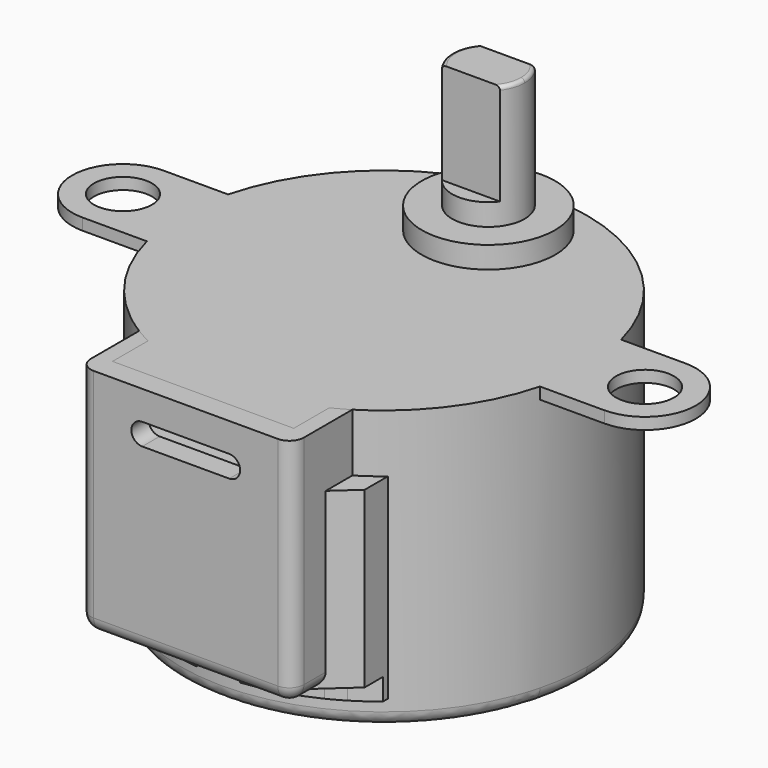
from build123d import *
from build123d import SkipClean  # not in build123d's __all__

# Parameters (mm, degrees)
F0_R      = 2
F0_R_2    = 4.6
F1_DEPTH  = 0.8
F2_DEPTH  = 19.3
F3_R      = 1
F4_DEPTH  = 1.5
F7_DEPTH  = 4
F8_DEPTH  = 12
F9_DEPTH  = 13.5
F11_R     = 1
F14_DEPTH = 3
F15_DEPTH = 3
F16_DEPTH = 10
F17_R     = 0.25


with BuildPart() as f1:
    # F0 (on Top) → F1 (new body)
    with BuildSketch(Plane.XY):
        with BuildLine():
            ThreePointArc((-13.5554417117, -3.5), (-14, 0), (-13.5554417117, 3.5))
            Line((-13.5554417117, 3.5), (-18, 3.5))
            ThreePointArc((-18, 3.5), (-21.5, 0), (-18, -3.5))
            Line((-18, -3.5), (-13.5554417117, -3.5))
        make_face()
        with Locations((-18, 0)):
            Circle(F0_R, mode=Mode.SUBTRACT)
        with BuildLine():
            ThreePointArc((13.5554417117, -3.5), (13.8884157477, -1.7640600948), (14, 0))
            ThreePointArc((14, 0), (13.8884157477, 1.7640600948), (13.5554417117, 3.5))
            ThreePointArc((13.5554417117, 3.5), (0, 14), (-13.5554417117, 3.5))
            ThreePointArc((-13.5554417117, 3.5), (-14, 0), (-13.5554417117, -3.5))
            ThreePointArc((-13.5554417117, -3.5), (-11.7352824288, -7.6343399398), (-8.6933517225, -10.9738614821))
            ThreePointArc((-8.6933517225, -10.9738614821), (-8.0354789523, -11.4643394056), (-7.35, -11.9154311714))
            ThreePointArc((-7.35, -11.9154311714), (-6.8068823867, -12.2338200156), (-6.25, -12.5274698164))
            ThreePointArc((-6.25, -12.5274698164), (-3.937003937, -13.4350288425), (-1.5, -13.9194109071))
            ThreePointArc((-1.5, -13.9194109071), (0, -14), (1.5, -13.9194109071))
            ThreePointArc((1.5, -13.9194109071), (3.937003937, -13.4350288425), (6.25, -12.5274698164))
            ThreePointArc((6.25, -12.5274698164), (6.8068823867, -12.2338200156), (7.35, -11.9154311714))
            ThreePointArc((7.35, -11.9154311714), (8.1473851159, -11.3850830376), (8.9066482775, -10.8014636259))
            ThreePointArc((8.9066482775, -10.8014636259), (11.8094967903, -7.5190282324), (13.5554417117, -3.5))
        make_face()
        with Locations((0, 9)):
            Circle(F0_R_2, mode=Mode.SUBTRACT)
        with BuildLine():
            ThreePointArc((13.5554417117, 3.5), (13.8884157477, 1.7640600948), (14, 0))
            ThreePointArc((14, 0), (13.8884157477, -1.7640600948), (13.5554417117, -3.5))
            Line((13.5554417117, -3.5), (18, -3.5))
            ThreePointArc((18, -3.5), (21.5, 0), (18, 3.5))
            Line((18, 3.5), (13.5554417117, 3.5))
        make_face()
        with Locations((18, 0)):
            Circle(F0_R, mode=Mode.SUBTRACT)
        with Locations((0, 9)):
            Circle(F0_R_2)
        with BuildLine():
            ThreePointArc((2, 10.5), (2.3717082451, 9.790569415), (2.5, 9))
            ThreePointArc((2.5, 9), (2.3717082451, 8.209430585), (2, 7.5))
            ThreePointArc((2, 7.5), (0, 6.5), (-2, 7.5))
            ThreePointArc((-2, 7.5), (-2.5, 9), (-2, 10.5))
            ThreePointArc((-2, 10.5), (0, 11.5), (2, 10.5))
        make_face(mode=Mode.SUBTRACT)
        with BuildLine():
            ThreePointArc((2, 7.5), (2.3717082451, 8.209430585), (2.5, 9))
            ThreePointArc((2.5, 9), (2.3717082451, 9.790569415), (2, 10.5))
            Line((2, 10.5), (-2, 10.5))
            ThreePointArc((-2, 10.5), (-2.5, 9), (-2, 7.5))
            Line((-2, 7.5), (2, 7.5))
        make_face()
        with BuildLine():
            ThreePointArc((-1.5, -13.9194109071), (-3.937003937, -13.4350288425), (-6.25, -12.5274698164))
            Line((-6.25, -12.5274698164), (-6.25, -12.9263565834))
            ThreePointArc((-6.25, -12.9263565834), (-3.9357520983, -13.8246688211), (-1.5, -14.3040642142))
            Line((-1.5, -14.3040642142), (-1.5, -13.9194109071))
        make_face()
        with BuildLine():
            Line((1.5, -14.3040642142), (1.5, -13.9194109071))
            ThreePointArc((1.5, -13.9194109071), (0, -14), (-1.5, -13.9194109071))
            Line((-1.5, -13.9194109071), (-1.5, -14.3040642142))
            ThreePointArc((-1.5, -14.3040642142), (-3.9357520983, -13.8246688211), (-6.25, -12.9263565834))
            Line((-6.25, -12.9263565834), (-6.25, -15.591))
            Line((-6.25, -15.591), (6.25, -15.591))
            Line((6.25, -15.591), (6.25, -12.9263565834))
            ThreePointArc((6.25, -12.9263565834), (3.9357520983, -13.8246688211), (1.5, -14.3040642142))
        make_face()
        with BuildLine():
            Line((1.5, -14.3040642142), (1.5, -13.9194109071))
            ThreePointArc((1.5, -13.9194109071), (0, -14), (-1.5, -13.9194109071))
            Line((-1.5, -13.9194109071), (-1.5, -14.3040642142))
            ThreePointArc((-1.5, -14.3040642142), (-3.9357520983, -13.8246688211), (-6.25, -12.9263565834))
            Line((-6.25, -12.9263565834), (-6.25, -15.591))
            Line((-6.25, -15.591), (6.25, -15.591))
            Line((6.25, -15.591), (6.25, -12.9263565834))
            ThreePointArc((6.25, -12.9263565834), (3.9357520983, -13.8246688211), (1.5, -14.3040642142))
        make_face()
        with BuildLine():
            Line((6.25, -12.9263565834), (6.25, -12.5274698164))
            ThreePointArc((6.25, -12.5274698164), (3.937003937, -13.4350288425), (1.5, -13.9194109071))
            Line((1.5, -13.9194109071), (1.5, -14.3040642142))
            ThreePointArc((1.5, -14.3040642142), (3.9357520983, -13.8246688211), (6.25, -12.9263565834))
        make_face()
        with BuildLine():
            Line((-2, 10.5), (2, 10.5))
            ThreePointArc((2, 10.5), (0, 11.5), (-2, 10.5))
        make_face()
        with BuildLine():
            ThreePointArc((-2, 7.5), (0, 6.5), (2, 7.5))
            Line((2, 7.5), (-2, 7.5))
        make_face()
    extrude(amount=-F1_DEPTH)

    # F0 (on Top) → F2 (join)
    with BuildSketch(Plane.XY):
        with BuildLine():
            ThreePointArc((13.5554417117, -3.5), (13.8884157477, -1.7640600948), (14, 0))
            ThreePointArc((14, 0), (13.8884157477, 1.7640600948), (13.5554417117, 3.5))
            ThreePointArc((13.5554417117, 3.5), (0, 14), (-13.5554417117, 3.5))
            ThreePointArc((-13.5554417117, 3.5), (-14, 0), (-13.5554417117, -3.5))
            ThreePointArc((-13.5554417117, -3.5), (-11.7352824288, -7.6343399398), (-8.6933517225, -10.9738614821))
            ThreePointArc((-8.6933517225, -10.9738614821), (-8.0354789523, -11.4643394056), (-7.35, -11.9154311714))
            ThreePointArc((-7.35, -11.9154311714), (-6.8068823867, -12.2338200156), (-6.25, -12.5274698164))
            ThreePointArc((-6.25, -12.5274698164), (-3.937003937, -13.4350288425), (-1.5, -13.9194109071))
            ThreePointArc((-1.5, -13.9194109071), (0, -14), (1.5, -13.9194109071))
            ThreePointArc((1.5, -13.9194109071), (3.937003937, -13.4350288425), (6.25, -12.5274698164))
            ThreePointArc((6.25, -12.5274698164), (6.8068823867, -12.2338200156), (7.35, -11.9154311714))
            ThreePointArc((7.35, -11.9154311714), (8.1473851159, -11.3850830376), (8.9066482775, -10.8014636259))
            ThreePointArc((8.9066482775, -10.8014636259), (11.8094967903, -7.5190282324), (13.5554417117, -3.5))
        make_face()
        with Locations((0, 9)):
            Circle(F0_R_2, mode=Mode.SUBTRACT)
        with Locations((0, 9)):
            Circle(F0_R_2)
        with BuildLine():
            ThreePointArc((2, 10.5), (2.3717082451, 9.790569415), (2.5, 9))
            ThreePointArc((2.5, 9), (2.3717082451, 8.209430585), (2, 7.5))
            ThreePointArc((2, 7.5), (0, 6.5), (-2, 7.5))
            ThreePointArc((-2, 7.5), (-2.5, 9), (-2, 10.5))
            ThreePointArc((-2, 10.5), (0, 11.5), (2, 10.5))
        make_face(mode=Mode.SUBTRACT)
        with BuildLine():
            ThreePointArc((2, 7.5), (2.3717082451, 8.209430585), (2.5, 9))
            ThreePointArc((2.5, 9), (2.3717082451, 9.790569415), (2, 10.5))
            Line((2, 10.5), (-2, 10.5))
            ThreePointArc((-2, 10.5), (-2.5, 9), (-2, 7.5))
            Line((-2, 7.5), (2, 7.5))
        make_face()
        with BuildLine():
            Line((-2, 10.5), (2, 10.5))
            ThreePointArc((2, 10.5), (0, 11.5), (-2, 10.5))
        make_face()
        with BuildLine():
            ThreePointArc((-2, 7.5), (0, 6.5), (2, 7.5))
            Line((2, 7.5), (-2, 7.5))
        make_face()
    extrude(amount=-F2_DEPTH)

    # F3
    f3_edges = [f1.edges().sort_by_distance(p)[0] for p in [
        (13.555442, 3.5, -19.3),
    ]]
    fillet(f3_edges, radius=F3_R)

    # F0 (on Top) → F4 (join)
    with BuildSketch(Plane.XY):
        with Locations((0, 9)):
            Circle(F0_R_2)
        with BuildLine():
            ThreePointArc((2, 10.5), (2.3717082451, 9.790569415), (2.5, 9))
            ThreePointArc((2.5, 9), (2.3717082451, 8.209430585), (2, 7.5))
            ThreePointArc((2, 7.5), (0, 6.5), (-2, 7.5))
            ThreePointArc((-2, 7.5), (-2.5, 9), (-2, 10.5))
            ThreePointArc((-2, 10.5), (0, 11.5), (2, 10.5))
        make_face(mode=Mode.SUBTRACT)
    extrude(amount=F4_DEPTH)


with BuildPart() as f7:
    # F6 (on offset) → F7 (new body)
    with BuildSketch(Plane.XY.offset(-4)):
        with BuildLine():
            ThreePointArc((-6.25, -12.9263565834), (-6.8067194333, -12.6362058443), (-7.35, -12.3216105412))
            Line((-7.35, -12.3216105412), (-7.35, -14.2114134505))
            Line((-7.35, -14.2114134505), (-7.35, -17.091))
            Line((-7.35, -17.091), (7.35, -17.091))
            Line((7.35, -17.091), (7.35, -14.2114134505))
            Line((7.35, -14.2114134505), (7.35, -12.3216105412))
            ThreePointArc((7.35, -12.3216105412), (6.8067194333, -12.6362058443), (6.25, -12.9263565834))
            Line((6.25, -12.9263565834), (6.25, -15.591))
            Line((6.25, -15.591), (-6.25, -15.591))
            Line((-6.25, -15.591), (-6.25, -12.9263565834))
        make_face()
        with BuildLine():
            ThreePointArc((-6.25, -12.5274698164), (-6.8068823867, -12.2338200156), (-7.35, -11.9154311714))
            Line((-7.35, -11.9154311714), (-7.35, -12.3216105412))
            ThreePointArc((-7.35, -12.3216105412), (-6.8067194333, -12.6362058443), (-6.25, -12.9263565834))
            Line((-6.25, -12.9263565834), (-6.25, -12.5274698164))
        make_face()
        with BuildLine():
            Line((7.35, -12.3216105412), (7.35, -11.9154311714))
            ThreePointArc((7.35, -11.9154311714), (6.8068823867, -12.2338200156), (6.25, -12.5274698164))
            Line((6.25, -12.5274698164), (6.25, -12.9263565834))
            ThreePointArc((6.25, -12.9263565834), (6.8067194333, -12.6362058443), (7.35, -12.3216105412))
        make_face()
    extrude(amount=F7_DEPTH)

    # F6 (on offset) → F8 (join)
    with BuildSketch(Plane.XY.offset(-4)):
        with BuildLine():
            ThreePointArc((-6.25, -12.9263565834), (-6.8067194333, -12.6362058443), (-7.35, -12.3216105412))
            Line((-7.35, -12.3216105412), (-7.35, -14.2114134505))
            Line((-7.35, -14.2114134505), (-7.35, -17.091))
            Line((-7.35, -17.091), (7.35, -17.091))
            Line((7.35, -17.091), (7.35, -14.2114134505))
            Line((7.35, -14.2114134505), (7.35, -12.3216105412))
            ThreePointArc((7.35, -12.3216105412), (6.8067194333, -12.6362058443), (6.25, -12.9263565834))
            Line((6.25, -12.9263565834), (6.25, -15.591))
            Line((6.25, -15.591), (-6.25, -15.591))
            Line((-6.25, -15.591), (-6.25, -12.9263565834))
        make_face()
        with BuildLine():
            ThreePointArc((-1.5, -13.9194109071), (-3.937003937, -13.4350288425), (-6.25, -12.5274698164))
            Line((-6.25, -12.5274698164), (-6.25, -12.9263565834))
            ThreePointArc((-6.25, -12.9263565834), (-3.9357520983, -13.8246688211), (-1.5, -14.3040642142))
            Line((-1.5, -14.3040642142), (-1.5, -13.9194109071))
        make_face()
        with BuildLine():
            ThreePointArc((-6.25, -12.5274698164), (-6.8068823867, -12.2338200156), (-7.35, -11.9154311714))
            Line((-7.35, -11.9154311714), (-7.35, -12.3216105412))
            ThreePointArc((-7.35, -12.3216105412), (-6.8067194333, -12.6362058443), (-6.25, -12.9263565834))
            Line((-6.25, -12.9263565834), (-6.25, -12.5274698164))
        make_face()
        with BuildLine():
            ThreePointArc((-7.35, -11.9154311714), (-8.0354789523, -11.4643394056), (-8.6933517225, -10.9738614821))
            Line((-8.6933517225, -10.9738614821), (-8.6933517225, -11.3928156516))
            ThreePointArc((-8.6933517225, -11.3928156516), (-8.0351072557, -11.876639438), (-7.35, -12.3216105412))
            Line((-7.35, -12.3216105412), (-7.35, -11.9154311714))
        make_face()
        with BuildLine():
            ThreePointArc((-7.35, -12.3216105412), (-8.0351072557, -11.876639438), (-8.6933517225, -11.3928156516))
            Line((-8.6933517225, -11.3928156516), (-8.6933517225, -12.9738614821))
            Line((-8.6933517225, -12.9738614821), (-7.35, -14.2114134505))
            Line((-7.35, -14.2114134505), (-7.35, -12.3216105412))
        make_face()
        with BuildLine():
            Line((7.35, -12.3216105412), (7.35, -11.9154311714))
            ThreePointArc((7.35, -11.9154311714), (6.8068823867, -12.2338200156), (6.25, -12.5274698164))
            Line((6.25, -12.5274698164), (6.25, -12.9263565834))
            ThreePointArc((6.25, -12.9263565834), (6.8067194333, -12.6362058443), (7.35, -12.3216105412))
        make_face()
        with BuildLine():
            Line((8.9066482775, -11.2229927703), (8.9066482775, -10.8014636259))
            ThreePointArc((8.9066482775, -10.8014636259), (8.1473851159, -11.3850830376), (7.35, -11.9154311714))
            Line((7.35, -11.9154311714), (7.35, -12.3216105412))
            ThreePointArc((7.35, -12.3216105412), (8.146864032, -11.7985711133), (8.9066482775, -11.2229927703))
        make_face()
        with BuildLine():
            Line((8.9066482775, -12.8014636259), (8.9066482775, -11.2229927703))
            ThreePointArc((8.9066482775, -11.2229927703), (8.146864032, -11.7985711133), (7.35, -12.3216105412))
            Line((7.35, -12.3216105412), (7.35, -14.2114134505))
            Line((7.35, -14.2114134505), (8.9066482775, -12.8014636259))
        make_face()
        with BuildLine():
            Line((6.25, -12.9263565834), (6.25, -12.5274698164))
            ThreePointArc((6.25, -12.5274698164), (3.937003937, -13.4350288425), (1.5, -13.9194109071))
            Line((1.5, -13.9194109071), (1.5, -14.3040642142))
            ThreePointArc((1.5, -14.3040642142), (3.9357520983, -13.8246688211), (6.25, -12.9263565834))
        make_face()
        with BuildLine():
            ThreePointArc((1.5, -13.9194109071), (0, -14), (-1.5, -13.9194109071))
            Line((-1.5, -13.9194109071), (-1.5, -14.3040642142))
            ThreePointArc((-1.5, -14.3040642142), (-3.9357520983, -13.8246688211), (-6.25, -12.9263565834))
            Line((-6.25, -12.9263565834), (-6.25, -15.591))
            Line((-6.25, -15.591), (6.25, -15.591))
            Line((6.25, -15.591), (6.25, -12.9263565834))
            ThreePointArc((6.25, -12.9263565834), (3.9357520983, -13.8246688211), (1.5, -14.3040642142))
            Line((1.5, -14.3040642142), (1.5, -13.9194109071))
        make_face()
    extrude(amount=-F8_DEPTH)

    # F6 (on offset) → F9 (join)
    with BuildSketch(Plane.XY.offset(-4)):
        with BuildLine():
            ThreePointArc((-7.35, -11.9154311714), (-8.0354789523, -11.4643394056), (-8.6933517225, -10.9738614821))
            Line((-8.6933517225, -10.9738614821), (-8.6933517225, -11.3928156516))
            ThreePointArc((-8.6933517225, -11.3928156516), (-8.0351072557, -11.876639438), (-7.35, -12.3216105412))
            Line((-7.35, -12.3216105412), (-7.35, -11.9154311714))
        make_face()
        with BuildLine():
            ThreePointArc((-6.25, -12.5274698164), (-6.8068823867, -12.2338200156), (-7.35, -11.9154311714))
            Line((-7.35, -11.9154311714), (-7.35, -12.3216105412))
            ThreePointArc((-7.35, -12.3216105412), (-6.8067194333, -12.6362058443), (-6.25, -12.9263565834))
            Line((-6.25, -12.9263565834), (-6.25, -12.5274698164))
        make_face()
        with BuildLine():
            ThreePointArc((-1.5, -13.9194109071), (-3.937003937, -13.4350288425), (-6.25, -12.5274698164))
            Line((-6.25, -12.5274698164), (-6.25, -12.9263565834))
            ThreePointArc((-6.25, -12.9263565834), (-3.9357520983, -13.8246688211), (-1.5, -14.3040642142))
            Line((-1.5, -14.3040642142), (-1.5, -13.9194109071))
        make_face()
        with BuildLine():
            Line((6.25, -12.9263565834), (6.25, -12.5274698164))
            ThreePointArc((6.25, -12.5274698164), (3.937003937, -13.4350288425), (1.5, -13.9194109071))
            Line((1.5, -13.9194109071), (1.5, -14.3040642142))
            ThreePointArc((1.5, -14.3040642142), (3.9357520983, -13.8246688211), (6.25, -12.9263565834))
        make_face()
        with BuildLine():
            Line((7.35, -12.3216105412), (7.35, -11.9154311714))
            ThreePointArc((7.35, -11.9154311714), (6.8068823867, -12.2338200156), (6.25, -12.5274698164))
            Line((6.25, -12.5274698164), (6.25, -12.9263565834))
            ThreePointArc((6.25, -12.9263565834), (6.8067194333, -12.6362058443), (7.35, -12.3216105412))
        make_face()
        with BuildLine():
            Line((8.9066482775, -11.2229927703), (8.9066482775, -10.8014636259))
            ThreePointArc((8.9066482775, -10.8014636259), (8.1473851159, -11.3850830376), (7.35, -11.9154311714))
            Line((7.35, -11.9154311714), (7.35, -12.3216105412))
            ThreePointArc((7.35, -12.3216105412), (8.146864032, -11.7985711133), (8.9066482775, -11.2229927703))
        make_face()
    extrude(amount=-F9_DEPTH)

    # F10: union 

    # F11
    f11_edges = [f7.edges().sort_by_distance(p)[0] for p in [
        (-7.35, -17.091, -8),
        (0, -17.091, -16),
        (7.35, -17.091, -8),
        (-7.35, -15.651207, -16),
        (7.35, -15.651207, -16),
    ]]
    fillet(f11_edges, radius=F11_R)

    # F13 (on offset) → F14 (cut)
    with BuildSketch(Plane.XZ.offset(17.091)):
        with BuildLine():
            ThreePointArc((3, -3.5), (3.75, -2.75), (3, -2))
            Line((3, -2), (-3, -2))
            ThreePointArc((-3, -2), (-3.75, -2.75), (-3, -3.5))
            Line((-3, -3.5), (3, -3.5))
        make_face()
    extrude(amount=-F14_DEPTH, mode=Mode.SUBTRACT)


with BuildPart() as f15:
    # F0 (on Top) → F15 (new body)
    with BuildSketch(Plane.XY):
        with BuildLine():
            Line((-2, 10.5), (2, 10.5))
            ThreePointArc((2, 10.5), (0, 11.5), (-2, 10.5))
        make_face()
        with BuildLine():
            ThreePointArc((2, 7.5), (2.3717082451, 8.209430585), (2.5, 9))
            ThreePointArc((2.5, 9), (2.3717082451, 9.790569415), (2, 10.5))
            Line((2, 10.5), (-2, 10.5))
            ThreePointArc((-2, 10.5), (-2.5, 9), (-2, 7.5))
            Line((-2, 7.5), (2, 7.5))
        make_face()
        with BuildLine():
            ThreePointArc((-2, 7.5), (0, 6.5), (2, 7.5))
            Line((2, 7.5), (-2, 7.5))
        make_face()
    extrude(amount=F15_DEPTH)

    # F0 (on Top) → F16 (join)
    with BuildSketch(Plane.XY):
        with BuildLine():
            ThreePointArc((2, 7.5), (2.3717082451, 8.209430585), (2.5, 9))
            ThreePointArc((2.5, 9), (2.3717082451, 9.790569415), (2, 10.5))
            Line((2, 10.5), (-2, 10.5))
            ThreePointArc((-2, 10.5), (-2.5, 9), (-2, 7.5))
            Line((-2, 7.5), (2, 7.5))
        make_face()
    with SkipClean():  # cleaning this boolean's faces spoils the solid; the shape is the same uncleaned
        extrude(amount=F16_DEPTH)

    # F17
    f17_edges = [f15.edges().sort_by_distance(p)[0] for p in [
        (2.5, 9, 10),
        (-2.5, 9, 10),
    ]]
    fillet(f17_edges, radius=F17_R)


solid = Compound([f1.part, f7.part, f15.part])
